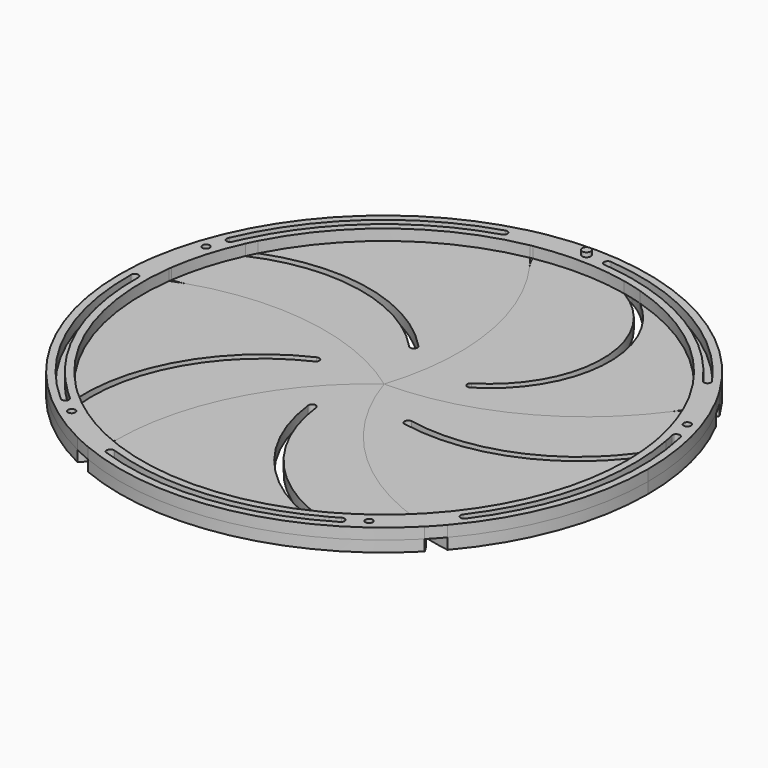
from build123d import *

# Parameters (mm, degrees)
F0_R     = 1.05
F1_DEPTH = 3.175
F2_DEPTH = 3.175
F3_DEPTH = 3.175
F4_DEPTH = 3.175
F5_DEPTH = 3.175
F6_DEPTH = 3.175
F7_R     = 1.05
F8_DEPTH = 25.4
F7_R_2   = 1.27
F9_DEPTH = 1.27


with BuildPart() as f1:
    # F0 (on Top) → F1 (new body)
    with BuildSketch(Plane.XY):
        with BuildLine():
            ThreePointArc((57.8988454356, -49.5395165219), (71.4784303906, -26.4059460899), (76.2, 0))
            ThreePointArc((76.2, 0), (74.0080436984, 18.1452326504), (67.5582816814, 35.2465399189))
            ThreePointArc((67.5582816814, 35.2465399189), (64.4660283996, 34.378247791), (61.6866117698, 32.7686500845))
            ThreePointArc((61.6866117698, 32.7686500846), (65.7907131471, 23.4649645981), (68.500497271, 13.6639808848))
            ThreePointArc((68.500497271, 13.6639808848), (69.3811022372, 15.2667591262), (70.201874573, 16.9009855397))
            ThreePointArc((70.201874573, 16.9009855397), (71.2638826106, 17.4908189825), (72.1717519503, 16.683640053))
            ThreePointArc((72.1717519503, 16.683640053), (72.2128589156, 16.5048063375), (72.2535227511, 16.3258713412))
            ThreePointArc((72.2535227511, 16.3258713412), (72.4179099959, -15.5804986063), (59.1463284149, -44.5961597006))
            ThreePointArc((59.1463284149, -44.5961597006), (57.6757970275, -44.802405764), (57.469550964, -43.3318743766))
            ThreePointArc((57.469550964, -43.3318743766), (70.0826247273, -16.3959243817), (70.727986059, 13.3398880445))
            ThreePointArc((70.727986059, 13.3398880445), (69.9127245645, 11.9184009517), (69.0527176616, 10.5235299949))
            ThreePointArc((69.0527176616, 10.5235299949), (69.6503942152, 5.2768442909), (69.85, 0))
            ThreePointArc((69.85, 0), (64.8935700225, -25.8427372725), (50.7276787478, -48.0179665215))
            ThreePointArc((50.7276787478, -48.0179665215), (54.2941569474, -48.8687853418), (57.8988454356, -49.5395165219))
        make_face()
        with Locations((69.4509021025, 22.5659660142)):
            Circle(F0_R, mode=Mode.SUBTRACT)
        with BuildLine():
            ThreePointArc((61.6866117698, 32.7686500845), (64.4660283996, 34.378247791), (67.5582816814, 35.2465399189))
            ThreePointArc((67.5582816814, 35.2465399189), (66.3207917987, 37.5232271425), (65.0066071965, 39.7565217391))
            ThreePointArc((65.0066071965, 39.7565217391), (63.2547939348, 36.5355265965), (61.3435147778, 33.4065217391))
            ThreePointArc((61.3435147778, 33.4065217391), (61.5158900581, 33.0880306208), (61.6866117698, 32.7686500846))
        make_face()
        with BuildLine():
            ThreePointArc((54.398108617, -53.359964195), (56.1809614325, -51.4795063352), (57.8988454356, -49.5395165219))
            ThreePointArc((57.8988454356, -49.5395165219), (54.2941569474, -48.8687853418), (50.7276787478, -48.0179665215))
            ThreePointArc((50.7276787478, -48.0179665215), (50.4780425853, -48.2803243232), (50.2270495554, -48.541384333))
            ThreePointArc((50.2270495554, -48.541384333), (52.6167549158, -50.6873735848), (54.398108617, -53.359964195))
        make_face()
        with BuildLine():
            ThreePointArc((61.3435147778, 33.4065217391), (63.2547939348, 36.5355265965), (65.0066071965, 39.7565217391))
            ThreePointArc((65.0066071965, 39.7565217391), (31.5990481128, 69.3393117817), (-12.6447943163, 75.1435238507))
            ThreePointArc((-12.6447943163, 75.1435238507), (-12.7745582452, 71.9342991933), (-12.1026268308, 68.7935238507))
            ThreePointArc((-12.1026268308, 68.7935238507), (1.2700549081, 69.8384525926), (14.5959016704, 68.3079948061))
            ThreePointArc((14.5959016704, 68.3079948061), (10.4665427153, 70.3209346952), (6.0938462702, 71.729145679))
            ThreePointArc((6.0938462702, 71.729145679), (5.3080441584, 72.9201009325), (6.4352132785, 73.7949432892))
            ThreePointArc((6.4352132785, 73.7949432892), (6.4752800387, 73.7914383477), (6.5153448899, 73.787911652))
            ThreePointArc((6.5153448899, 73.787911652), (37.0723258817, 64.1307124452), (60.69068892, 42.4705298226))
            ThreePointArc((60.69068892, 42.4705298226), (60.4324213932, 41.0082378256), (58.9701293962, 41.2665053524))
            ThreePointArc((58.9701293962, 41.2665053524), (39.869860882, 59.9232410526), (15.2829537028, 70.3337184508))
            ThreePointArc((15.2829537028, 70.3337184508), (17.9297919561, 68.6829049595), (20.4165739668, 66.799595863))
            ThreePointArc((20.4165739668, 66.799595863), (44.1582651124, 54.1208843448), (61.3435147778, 33.4065217391))
        make_face()
        with Locations((0, 73.025)):
            Circle(F0_R, mode=Mode.SUBTRACT)
        with BuildLine():
            ThreePointArc((-29.223152808, -70.3736267359), (15.1924579401, -74.6701360769), (54.398108617, -53.359964195))
            ThreePointArc((54.398108617, -53.359964195), (52.6167549158, -50.6873735848), (50.2270495554, -48.541384333))
            ThreePointArc((50.2270495554, -48.541384333), (42.6469559202, -55.3196136171), (34.1630358389, -60.9254419948))
            ThreePointArc((34.1630358389, -60.9254419949), (35.9594904295, -61.2676613714), (37.7673647093, -61.5432585154))
            ThreePointArc((37.7673647093, -61.5432585154), (38.6565081805, -62.3710196222), (38.1693824544, -63.4838866804))
            ThreePointArc((38.1693824544, -63.4838866804), (38.0120042348, -63.5782443848), (37.8543927568, -63.6722119453))
            ThreePointArc((37.8543927568, -63.6722119453), (7.5604301592, -73.6881640483), (-24.1362476499, -70.0324722852))
            ThreePointArc((-24.1362476499, -70.0324722852), (-24.7868185019, -68.6976473655), (-23.4519935822, -68.0470765134))
            ThreePointArc((-23.4519935822, -68.0470765134), (6.0632713273, -71.7191561984), (34.5431371215, -63.144059917))
            ThreePointArc((34.5431371215, -63.144059917), (32.9392929024, -62.8079638292), (31.3469350413, -62.4210874907))
            ThreePointArc((31.3469350413, -62.4210874907), (0.7540037914, -69.8459302915), (-29.9920851413, -63.0832571201))
            ThreePointArc((-29.9920851413, -63.0832571201), (-29.6991595508, -66.7380969266), (-29.223152808, -70.3736267359))
        make_face()
        with Locations((42.9230180487, -59.0784660142)):
            Circle(F0_R, mode=Mode.SUBTRACT)
        with BuildLine():
            ThreePointArc((-12.1026268308, 68.7935238507), (-12.7745582452, 71.9342991933), (-12.6447943163, 75.1435238507))
            ThreePointArc((-12.6447943163, 75.1435238507), (-15.1924579401, 74.6701360769), (-17.7225526948, 74.1103982311))
            ThreePointArc((-17.7225526948, 74.1103982311), (-15.2005443443, 71.4489825753), (-12.8153016257, 68.6643324022))
            ThreePointArc((-12.8153016257, 68.6643324022), (-12.4591316812, 68.7298518677), (-12.1026268308, 68.7935238507))
        make_face()
        with BuildLine():
            ThreePointArc((-33.9384016324, -68.2248114298), (-31.5990481128, -69.3393117817), (-29.223152808, -70.3736267359))
            ThreePointArc((-29.223152808, -70.3736267359), (-29.6991595508, -66.7380969266), (-29.9920851413, -63.0832571201))
            ThreePointArc((-29.9920851413, -63.0832571201), (-30.3187440548, -62.9269120404), (-30.6445879899, -62.7688754633))
            ThreePointArc((-30.6445879899, -62.7688754633), (-31.9470854839, -65.7047674669), (-33.9384016324, -68.2248114298))
        make_face()
        with BuildLine():
            ThreePointArc((-12.8153016257, 68.6643324022), (-15.2005443443, 71.4489825753), (-17.7225526948, 74.1103982311))
            ThreePointArc((-17.7225526948, 74.1103982311), (-56.1809614325, 51.4795063352), (-75.3731943497, 11.1947118553))
            ThreePointArc((-75.3731943497, 11.1947118553), (-72.3611395863, 10.0795940673), (-69.1664465044, 9.748085861))
            ThreePointArc((-69.1664465044, 9.748085861), (-67.0181651444, 19.6872557934), (-63.4495528671, 29.209189324))
            ThreePointArc((-63.4495528671, 29.209189324), (-65.1040666631, 28.4301211007), (-66.728659616, 27.590442034))
            ThreePointArc((-66.728659616, 27.590442034), (-67.9345375656, 27.7374894172), (-68.1945714194, 28.9241430976))
            ThreePointArc((-68.1945714194, 28.9241430976), (-68.1227118322, 29.0929846806), (-68.0504342143, 29.2616477363))
            ThreePointArc((-68.0504342143, 29.2616477363), (-49.4293325796, 55.1710676508), (-21.6374198617, 70.8443906511))
            ThreePointArc((-21.6374198617, 70.8443906511), (-20.3892075809, 70.305014085), (-20.7199588174, 68.9860885383))
            ThreePointArc((-20.7199588174, 68.9860885383), (-20.7480884716, 68.9666575811), (-20.7768358082, 68.948152712))
            ThreePointArc((-20.7768358082, 68.948152712), (-20.8967811774, 68.8840443635), (-21.0240066762, 68.8359772813))
            ThreePointArc((-21.0240066762, 68.8359772813), (-47.0607518656, 54.4581147199), (-65.0611321594, 30.7806709988))
            ThreePointArc((-65.0611321594, 30.7806709988), (-63.5660426061, 31.451479531), (-62.050397829, 32.0744544655))
            ThreePointArc((-62.050397829, 32.0744544655), (-41.664409639, 56.063352285), (-12.8153016257, 68.6643324022))
        make_face()
        with Locations((-69.4509021025, 22.5659660142)):
            Circle(F0_R, mode=Mode.SUBTRACT)
        with BuildLine():
            ThreePointArc((-75.9597471294, 6.0462232875), (-66.3207917987, -37.5232271425), (-33.9384016324, -68.2248114298))
            ThreePointArc((-33.9384016324, -68.2248114298), (-31.9470854839, -65.7047674669), (-30.6445879899, -62.7688754633))
            ThreePointArc((-30.6445879899, -62.7688754633), (-39.4334448718, -57.654366058), (-47.3865799637, -51.3179748173))
            ThreePointArc((-47.3865799637, -51.3179748173), (-47.1569149337, -53.132256265), (-46.8603595171, -54.9368110806))
            ThreePointArc((-46.8603595171, -54.9368110806), (-47.3728466687, -56.038229022), (-48.5817762639, -55.9188397594))
            ThreePointArc((-48.5817762639, -55.9188397594), (-48.720148318, -55.7983223123), (-48.8582214039, -55.6774624623))
            ThreePointArc((-48.8582214039, -55.6774624623), (-67.745307188, -29.9612913441), (-74.0633498234, 1.3137115121))
            ThreePointArc((-74.0633498234, 1.3137115121), (-72.9948933347, 2.344924745), (-71.9636801018, 1.2764682563))
            ThreePointArc((-71.9636801018, 1.2764682563), (-66.335316964, -27.9289517934), (-49.3791532399, -52.3650632608))
            ThreePointArc((-49.3791532399, -52.3650632608), (-49.5551219855, -50.7358573623), (-49.6792463629, -49.1018836789))
            ThreePointArc((-49.6792463629, -49.1018836789), (-66.1944271551, -22.3006796671), (-69.2638067586, 9.0303695003))
            ThreePointArc((-69.2638067586, 9.0303695003), (-72.6492469871, 7.6223730967), (-75.9597471294, 6.0462232875))
        make_face()
        with Locations((-42.9230180487, -59.0784660142)):
            Circle(F0_R, mode=Mode.SUBTRACT)
        with BuildLine():
            ThreePointArc((-69.1664465044, 9.748085861), (-72.3611395863, 10.0795940673), (-75.3731943497, 11.1947118553))
            ThreePointArc((-75.3731943497, 11.1947118553), (-75.7102471784, 8.6254548976), (-75.9597471294, 6.0462232875))
            ThreePointArc((-75.9597471294, 6.0462232875), (-72.6492469871, 7.6223730967), (-69.2638067586, 9.0303695003))
            ThreePointArc((-69.2638067586, 9.0303695003), (-69.2160569074, 9.3893538752), (-69.1664465044, 9.748085861))
        make_face()
        with BuildLine():
            ThreePointArc((-63.4495528671, 29.209189324), (-62.7663272963, 30.649806814), (-62.050397829, 32.0744544655))
            ThreePointArc((-62.050397829, 32.0744544655), (-63.5660426061, 31.451479531), (-65.0611321594, 30.7806709988))
            ThreePointArc((-65.0611321594, 30.7806709988), (-65.6748421089, 29.4485269405), (-66.2612794858, 28.1041538906))
            ThreePointArc((-66.2612794858, 28.1041538906), (-66.4512663757, 27.8075363811), (-66.728659616, 27.590442034))
            ThreePointArc((-66.728659616, 27.590442034), (-65.1040666631, 28.4301211007), (-63.4495528671, 29.209189324))
        make_face()
        with BuildLine():
            ThreePointArc((14.5959016704, 68.3079948061), (17.5224764061, 67.6164574686), (20.4165739668, 66.799595863))
            ThreePointArc((20.4165739668, 66.799595863), (17.9297919561, 68.6829049595), (15.2829537028, 70.3337184508))
            ThreePointArc((15.2829537028, 70.3337184508), (10.7896051737, 71.1616824225), (6.2527772625, 71.7028827977))
            ThreePointArc((6.2527772625, 71.7028827977), (6.1728073816, 71.7129619314), (6.0938462702, 71.729145679))
            ThreePointArc((6.0938462702, 71.729145679), (10.4665427153, 70.3209346952), (14.5959016704, 68.3079948061))
        make_face()
        with BuildLine():
            ThreePointArc((70.201874573, 16.9009855397), (69.3811022372, 15.2667591262), (68.500497271, 13.6639808848))
            ThreePointArc((68.500497271, 13.6639808848), (68.7945298881, 12.0969069385), (69.0527176616, 10.5235299949))
            ThreePointArc((69.0527176616, 10.5235299949), (69.9127245645, 11.9184009517), (70.727986059, 13.3398880445))
            ThreePointArc((70.727986059, 13.3398880445), (70.4414732064, 14.7783448841), (70.1257083581, 16.2106647697))
            ThreePointArc((70.1257083581, 16.2106647697), (70.105063583, 16.5623048678), (70.201874573, 16.9009855397))
        make_face()
        with BuildLine():
            ThreePointArc((37.7673647093, -61.5432585154), (35.9594904295, -61.2676613714), (34.1630358389, -60.9254419949))
            ThreePointArc((34.1630358389, -60.9254419948), (32.7635210263, -61.6893361121), (31.3469350413, -62.4210874907))
            ThreePointArc((31.3469350413, -62.4210874907), (32.9392929024, -62.8079638292), (34.5431371215, -63.144059917))
            ThreePointArc((34.5431371215, -63.144059917), (35.8226535316, -62.4270623925), (37.0872939879, -61.6841409898))
            ThreePointArc((37.0872939879, -61.6841409898), (37.4153440082, -61.5558438758), (37.7673647093, -61.5432585154))
        make_face()
        with BuildLine():
            ThreePointArc((-46.8603595171, -54.9368110806), (-47.1569149337, -53.132256265), (-47.3865799637, -51.3179748173))
            ThreePointArc((-47.3865799637, -51.3179748173), (-48.5455603027, -50.2230133992), (-49.6792463629, -49.1018836789))
            ThreePointArc((-49.6792463629, -49.1018836789), (-49.5551219855, -50.7358573623), (-49.3791532399, -52.3650632608))
            ThreePointArc((-49.3791532399, -52.3650632608), (-48.3018557566, -53.3603912604), (-47.2045001228, -54.3335604683))
            ThreePointArc((-47.2045001228, -54.3335604683), (-46.9811092852, -54.6059085892), (-46.8603595171, -54.9368110806))
        make_face()
    extrude(amount=F1_DEPTH)


with BuildPart() as f2:
    # F0 (on Top) → F2 (new body)
    with BuildSketch(Plane.XY):
        with BuildLine():
            ThreePointArc((61.3435147778, 33.4065217391), (63.2547939348, 36.5355265965), (65.0066071965, 39.7565217391))
            ThreePointArc((65.0066071965, 39.7565217391), (31.5990481128, 69.3393117817), (-12.6447943163, 75.1435238507))
            ThreePointArc((-12.6447943163, 75.1435238507), (-12.7745582452, 71.9342991933), (-12.1026268308, 68.7935238507))
            ThreePointArc((-12.1026268308, 68.7935238507), (1.2700549081, 69.8384525926), (14.5959016704, 68.3079948061))
            ThreePointArc((14.5959016704, 68.3079948061), (10.4665427153, 70.3209346952), (6.0938462702, 71.729145679))
            ThreePointArc((6.0938462702, 71.729145679), (5.3080441584, 72.9201009325), (6.4352132785, 73.7949432892))
            ThreePointArc((6.4352132785, 73.7949432892), (6.4752800387, 73.7914383477), (6.5153448899, 73.787911652))
            ThreePointArc((6.5153448899, 73.787911652), (37.0723258817, 64.1307124452), (60.69068892, 42.4705298226))
            ThreePointArc((60.69068892, 42.4705298226), (60.4324213932, 41.0082378256), (58.9701293962, 41.2665053524))
            ThreePointArc((58.9701293962, 41.2665053524), (39.869860882, 59.9232410526), (15.2829537028, 70.3337184508))
            ThreePointArc((15.2829537028, 70.3337184508), (17.9297919561, 68.6829049595), (20.4165739668, 66.799595863))
            ThreePointArc((20.4165739668, 66.799595863), (44.1582651124, 54.1208843448), (61.3435147778, 33.4065217391))
        make_face()
        with Locations((0, 73.025)):
            Circle(F0_R, mode=Mode.SUBTRACT)
        with BuildLine():
            ThreePointArc((59.0784660142, 30.1019819513), (60.2336563747, 31.7387157796), (61.3435147778, 33.4065217391))
            ThreePointArc((61.3435147778, 33.4065217391), (44.1582651124, 54.1208843448), (20.4165739668, 66.799595863))
            ThreePointArc((20.4165739668, 66.799595863), (32.7606539852, 37.7278540517), (16.2490976022, 10.8036829548))
            ThreePointArc((16.2490976022, 10.8036829548), (14.9772255674, 10.9446710874), (14.7861444758, 12.2099869147))
            ThreePointArc((14.7861444758, 12.2099869147), (14.9479136837, 12.4293059965), (15.160676558, 12.5996060128))
            ThreePointArc((15.160676558, 12.5996060128), (30.7540739017, 40.6147500395), (14.5959016704, 68.3079948061))
            ThreePointArc((14.5959016704, 68.3079948061), (1.2700549081, 69.8384525926), (-12.1026268308, 68.7935238507))
            ThreePointArc((-12.1026268308, 68.7935238507), (-11.3583497528, 67.0779959221), (-10.3724360882, 65.4889840629))
            ThreePointArc((-10.3724360882, 65.4889840629), (2.6750389695, 33.9895928238), (0, 0))
            ThreePointArc((0, 0), (33.1526562435, 7.9592485711), (59.0784660142, 30.1019819513))
        make_face()
        with BuildLine():
            ThreePointArc((6.5941442709, 73.7686804079), (11.055453508, 72.3469119056), (15.2829537028, 70.3337184508))
            ThreePointArc((15.2829537028, 70.3337184508), (39.869860882, 59.9232410526), (58.9701293962, 41.2665053524))
            ThreePointArc((58.9701293962, 41.2665053524), (60.4324213932, 41.0082378256), (60.69068892, 42.4705298226))
            ThreePointArc((60.69068892, 42.4705298226), (37.0723258817, 64.1307124452), (6.5153448899, 73.787911652))
            ThreePointArc((6.5153448899, 73.787911652), (6.5547502363, 73.7783192049), (6.5941442709, 73.7686804079))
        make_face()
    extrude(amount=-F2_DEPTH)


with BuildPart() as f2b:
    # F0 (on Top) → F2, piece 2 (new body)
    with BuildSketch(Plane.XY):
        with BuildLine():
            ThreePointArc((34.1630358389, -60.9254419948), (42.6469559202, -55.3196136171), (50.2270495554, -48.541384333))
            ThreePointArc((50.2270495554, -48.541384333), (48.6165547344, -47.5909681745), (46.8849360882, -46.8849360882))
            ThreePointArc((46.8849360882, -46.8849360882), (17.8144294063, -29.0705066819), (0, 0))
            ThreePointArc((0, 0), (-22.1427333802, -25.9258097708), (-30.1019819513, -59.0784660142))
            ThreePointArc((-30.1019819513, -59.0784660142), (-30.0745025786, -61.081615354), (-29.9920851413, -63.0832571201))
            ThreePointArc((-29.9920851413, -63.0832571201), (0.7540037914, -69.8459302915), (31.3469350413, -62.4210874907))
            ThreePointArc((31.3469350413, -62.4210874907), (5.5340708198, -46.501418093), (-6.8695410517, -18.826695952))
            ThreePointArc((-6.8695410517, -18.826695952), (-5.9562321753, -17.6558556998), (-4.7853919231, -18.5691645763))
            ThreePointArc((-4.7853919231, -18.5691645763), (7.8982881897, -45.9914925783), (34.1630358389, -60.9254419949))
        make_face()
    extrude(amount=-F2_DEPTH)

    # F0 (on Top) → F6 (join)
    with BuildSketch(Plane.XY):
        with BuildLine():
            ThreePointArc((37.8543927568, -63.6722119453), (36.1944718192, -63.4350516997), (34.5431371215, -63.144059917))
            ThreePointArc((34.5431371215, -63.144059917), (6.0632713273, -71.7191561984), (-23.4519935822, -68.0470765134))
            ThreePointArc((-23.4519935822, -68.0470765134), (-24.7868185019, -68.6976473655), (-24.1362476499, -70.0324722852))
            ThreePointArc((-24.1362476499, -70.0324722852), (7.5604301592, -73.6881640483), (37.8543927568, -63.6722119453))
        make_face()
        with BuildLine():
            ThreePointArc((-29.223152808, -70.3736267359), (15.1924579401, -74.6701360769), (54.398108617, -53.359964195))
            ThreePointArc((54.398108617, -53.359964195), (52.6167549158, -50.6873735848), (50.2270495554, -48.541384333))
            ThreePointArc((50.2270495554, -48.541384333), (42.6469559202, -55.3196136171), (34.1630358389, -60.9254419948))
            ThreePointArc((34.1630358389, -60.9254419949), (35.9594904295, -61.2676613714), (37.7673647093, -61.5432585154))
            ThreePointArc((37.7673647093, -61.5432585154), (38.6565081805, -62.3710196222), (38.1693824544, -63.4838866804))
            ThreePointArc((38.1693824544, -63.4838866804), (38.0120042348, -63.5782443848), (37.8543927568, -63.6722119453))
            ThreePointArc((37.8543927568, -63.6722119453), (7.5604301592, -73.6881640483), (-24.1362476499, -70.0324722852))
            ThreePointArc((-24.1362476499, -70.0324722852), (-24.7868185019, -68.6976473655), (-23.4519935822, -68.0470765134))
            ThreePointArc((-23.4519935822, -68.0470765134), (6.0632713273, -71.7191561984), (34.5431371215, -63.144059917))
            ThreePointArc((34.5431371215, -63.144059917), (32.9392929024, -62.8079638292), (31.3469350413, -62.4210874907))
            ThreePointArc((31.3469350413, -62.4210874907), (0.7540037914, -69.8459302915), (-29.9920851413, -63.0832571201))
            ThreePointArc((-29.9920851413, -63.0832571201), (-29.6991595508, -66.7380969266), (-29.223152808, -70.3736267359))
        make_face()
        with Locations((42.9230180487, -59.0784660142)):
            Circle(F0_R, mode=Mode.SUBTRACT)
        with BuildLine():
            ThreePointArc((34.1630358389, -60.9254419948), (42.6469559202, -55.3196136171), (50.2270495554, -48.541384333))
            ThreePointArc((50.2270495554, -48.541384333), (48.6165547344, -47.5909681745), (46.8849360882, -46.8849360882))
            ThreePointArc((46.8849360882, -46.8849360882), (17.8144294063, -29.0705066819), (0, 0))
            ThreePointArc((0, 0), (-22.1427333802, -25.9258097708), (-30.1019819513, -59.0784660142))
            ThreePointArc((-30.1019819513, -59.0784660142), (-30.0745025786, -61.081615354), (-29.9920851413, -63.0832571201))
            ThreePointArc((-29.9920851413, -63.0832571201), (0.7540037914, -69.8459302915), (31.3469350413, -62.4210874907))
            ThreePointArc((31.3469350413, -62.4210874907), (5.5340708198, -46.501418093), (-6.8695410517, -18.826695952))
            ThreePointArc((-6.8695410517, -18.826695952), (-5.9562321753, -17.6558556998), (-4.7853919231, -18.5691645763))
            ThreePointArc((-4.7853919231, -18.5691645763), (7.8982881897, -45.9914925783), (34.1630358389, -60.9254419949))
        make_face()
    extrude(amount=-F6_DEPTH)


with BuildPart() as f3:
    # F0 (on Top) → F3 (new body)
    with BuildSketch(Plane.XY):
        with BuildLine():
            ThreePointArc((68.500497271, 13.6639808848), (65.7907131471, 23.4649645981), (61.6866117698, 32.7686500846))
            ThreePointArc((61.6866117698, 32.7686500845), (60.2850420201, 31.5306732353), (59.0784660142, 30.1019819513))
            ThreePointArc((59.0784660142, 30.1019819513), (33.1526562435, 7.9592485711), (0, 0))
            ThreePointArc((0, 0), (17.8144294063, -29.0705066819), (46.8849360882, -46.8849360882))
            ThreePointArc((46.8849360882, -46.8849360882), (48.7985359141, -47.47780884), (50.7276787478, -48.0179665215))
            ThreePointArc((50.7276787478, -48.0179665215), (64.8935700225, -25.8427372725), (69.85, 0))
            ThreePointArc((69.85, 0), (69.6503942152, 5.2768442909), (69.0527176616, 10.5235299949))
            ThreePointArc((69.0527176616, 10.5235299949), (45.9355986257, -9.1065143384), (15.7824469369, -12.3510907783))
            ThreePointArc((15.7824469369, -12.3510907783), (14.9511396494, -11.1206728843), (16.1815575434, -10.2893655969))
            ThreePointArc((16.1815575434, -10.2893655969), (46.1812139878, -6.700434353), (68.500497271, 13.6639808848))
        make_face()
        with BuildLine():
            ThreePointArc((57.8988454356, -49.5395165219), (71.4784303906, -26.4059460899), (76.2, 0))
            ThreePointArc((76.2, 0), (74.0080436984, 18.1452326504), (67.5582816814, 35.2465399189))
            ThreePointArc((67.5582816814, 35.2465399189), (64.4660283996, 34.378247791), (61.6866117698, 32.7686500845))
            ThreePointArc((61.6866117698, 32.7686500846), (65.7907131471, 23.4649645981), (68.500497271, 13.6639808848))
            ThreePointArc((68.500497271, 13.6639808848), (69.3811022372, 15.2667591262), (70.201874573, 16.9009855397))
            ThreePointArc((70.201874573, 16.9009855397), (71.2638826106, 17.4908189825), (72.1717519503, 16.683640053))
            ThreePointArc((72.1717519503, 16.683640053), (72.2128589156, 16.5048063375), (72.2535227511, 16.3258713412))
            ThreePointArc((72.2535227511, 16.3258713412), (72.4179099959, -15.5804986063), (59.1463284149, -44.5961597006))
            ThreePointArc((59.1463284149, -44.5961597006), (57.6757970275, -44.802405764), (57.469550964, -43.3318743766))
            ThreePointArc((57.469550964, -43.3318743766), (70.0826247273, -16.3959243817), (70.727986059, 13.3398880445))
            ThreePointArc((70.727986059, 13.3398880445), (69.9127245645, 11.9184009517), (69.0527176616, 10.5235299949))
            ThreePointArc((69.0527176616, 10.5235299949), (69.6503942152, 5.2768442909), (69.85, 0))
            ThreePointArc((69.85, 0), (64.8935700225, -25.8427372725), (50.7276787478, -48.0179665215))
            ThreePointArc((50.7276787478, -48.0179665215), (54.2941569474, -48.8687853418), (57.8988454356, -49.5395165219))
        make_face()
        with Locations((69.4509021025, 22.5659660142)):
            Circle(F0_R, mode=Mode.SUBTRACT)
        with BuildLine():
            ThreePointArc((72.2535227511, 16.3258713412), (71.5150261751, 14.8204792632), (70.727986059, 13.3398880445))
            ThreePointArc((70.727986059, 13.3398880445), (70.0826247273, -16.3959243817), (57.469550964, -43.3318743766))
            ThreePointArc((57.469550964, -43.3318743766), (57.6757970275, -44.802405764), (59.1463284149, -44.5961597006))
            ThreePointArc((59.1463284149, -44.5961597006), (72.4179099959, -15.5804986063), (72.2535227511, 16.3258713412))
        make_face()
    extrude(amount=-F3_DEPTH)


with BuildPart() as f4:
    # F0 (on Top) → F4 (new body)
    with BuildSketch(Plane.XY):
        with BuildLine():
            ThreePointArc((-68.0504342143, 29.2616477363), (-66.5681306716, 30.0454581143), (-65.0611321594, 30.7806709988))
            ThreePointArc((-65.0611321594, 30.7806709988), (-47.0607518656, 54.4581147199), (-21.0240066762, 68.8359772813))
            ThreePointArc((-21.0240066762, 68.8359772813), (-20.8967811774, 68.8840443635), (-20.7768358082, 68.948152712))
            ThreePointArc((-20.7768358082, 68.948152712), (-20.7484067167, 68.9671347244), (-20.7199588174, 68.9860885383))
            ThreePointArc((-20.7199588174, 68.9860885383), (-20.3892075809, 70.305014085), (-21.6374198617, 70.8443906511))
            ThreePointArc((-21.6374198617, 70.8443906511), (-49.4293325796, 55.1710676508), (-68.0504342143, 29.2616477363))
        make_face()
        with BuildLine():
            ThreePointArc((-12.8153016257, 68.6643324022), (-15.2005443443, 71.4489825753), (-17.7225526948, 74.1103982311))
            ThreePointArc((-17.7225526948, 74.1103982311), (-56.1809614325, 51.4795063352), (-75.3731943497, 11.1947118553))
            ThreePointArc((-75.3731943497, 11.1947118553), (-72.3611395863, 10.0795940673), (-69.1664465044, 9.748085861))
            ThreePointArc((-69.1664465044, 9.748085861), (-67.0181651444, 19.6872557934), (-63.4495528671, 29.209189324))
            ThreePointArc((-63.4495528671, 29.209189324), (-65.1040666631, 28.4301211007), (-66.728659616, 27.590442034))
            ThreePointArc((-66.728659616, 27.590442034), (-67.9345375656, 27.7374894172), (-68.1945714194, 28.9241430976))
            ThreePointArc((-68.1945714194, 28.9241430976), (-68.1227118322, 29.0929846806), (-68.0504342143, 29.2616477363))
            ThreePointArc((-68.0504342143, 29.2616477363), (-49.4293325796, 55.1710676508), (-21.6374198617, 70.8443906511))
            ThreePointArc((-21.6374198617, 70.8443906511), (-20.3892075809, 70.305014085), (-20.7199588174, 68.9860885383))
            ThreePointArc((-20.7199588174, 68.9860885383), (-20.7480884716, 68.9666575811), (-20.7768358082, 68.948152712))
            ThreePointArc((-20.7768358082, 68.948152712), (-20.8967811774, 68.8840443635), (-21.0240066762, 68.8359772813))
            ThreePointArc((-21.0240066762, 68.8359772813), (-47.0607518656, 54.4581147199), (-65.0611321594, 30.7806709988))
            ThreePointArc((-65.0611321594, 30.7806709988), (-63.5660426061, 31.451479531), (-62.050397829, 32.0744544655))
            ThreePointArc((-62.050397829, 32.0744544655), (-41.664409639, 56.063352285), (-12.8153016257, 68.6643324022))
        make_face()
        with Locations((-69.4509021025, 22.5659660142)):
            Circle(F0_R, mode=Mode.SUBTRACT)
        with BuildLine():
            ThreePointArc((-65.4889840629, 10.3724360882), (-31.4993912391, 13.0474750577), (0, 0))
            ThreePointArc((0, 0), (2.6750389695, 33.9895928238), (-10.3724360882, 65.4889840629))
            ThreePointArc((-10.3724360882, 65.4889840629), (-11.5720890079, 67.093413951), (-12.8153016257, 68.6643324022))
            ThreePointArc((-12.8153016257, 68.6643324022), (-41.664409639, 56.063352285), (-62.050397829, 32.0744544655))
            ThreePointArc((-62.050397829, 32.0744544655), (-31.8100051071, 34.3675922868), (-5.5084787756, 19.2689318933))
            ThreePointArc((-5.5084787756, 19.2689318933), (-5.5591585447, 17.7848727432), (-7.0432176948, 17.8355525124))
            ThreePointArc((-7.0432176948, 17.8355525124), (-33.4229704404, 32.5654017762), (-63.4495528671, 29.209189324))
            ThreePointArc((-63.4495528671, 29.209189324), (-67.0181651444, 19.6872557934), (-69.1664465044, 9.748085861))
            ThreePointArc((-69.1664465044, 9.748085861), (-67.3048882234, 9.9258081418), (-65.4889840629, 10.3724360882))
        make_face()
    extrude(amount=-F4_DEPTH)


with BuildPart() as f5:
    # F0 (on Top) → F5 (new body)
    with BuildSketch(Plane.XY):
        with BuildLine():
            ThreePointArc((-48.8582214039, -55.6774624623), (-49.145612386, -54.0254972917), (-49.3791532399, -52.3650632608))
            ThreePointArc((-49.3791532399, -52.3650632608), (-66.335316964, -27.9289517934), (-71.9636801018, 1.2764682563))
            ThreePointArc((-71.9636801018, 1.2764682563), (-72.9948933347, 2.344924745), (-74.0633498234, 1.3137115121))
            ThreePointArc((-74.0633498234, 1.3137115121), (-67.745307188, -29.9612913441), (-48.8582214039, -55.6774624623))
        make_face()
        with BuildLine():
            ThreePointArc((-75.9597471294, 6.0462232875), (-66.3207917987, -37.5232271425), (-33.9384016324, -68.2248114298))
            ThreePointArc((-33.9384016324, -68.2248114298), (-31.9470854839, -65.7047674669), (-30.6445879899, -62.7688754633))
            ThreePointArc((-30.6445879899, -62.7688754633), (-39.4334448718, -57.654366058), (-47.3865799637, -51.3179748173))
            ThreePointArc((-47.3865799637, -51.3179748173), (-47.1569149337, -53.132256265), (-46.8603595171, -54.9368110806))
            ThreePointArc((-46.8603595171, -54.9368110806), (-47.3728466687, -56.038229022), (-48.5817762639, -55.9188397594))
            ThreePointArc((-48.5817762639, -55.9188397594), (-48.720148318, -55.7983223123), (-48.8582214039, -55.6774624623))
            ThreePointArc((-48.8582214039, -55.6774624623), (-67.745307188, -29.9612913441), (-74.0633498234, 1.3137115121))
            ThreePointArc((-74.0633498234, 1.3137115121), (-72.9948933347, 2.344924745), (-71.9636801018, 1.2764682563))
            ThreePointArc((-71.9636801018, 1.2764682563), (-66.335316964, -27.9289517934), (-49.3791532399, -52.3650632608))
            ThreePointArc((-49.3791532399, -52.3650632608), (-49.5551219855, -50.7358573623), (-49.6792463629, -49.1018836789))
            ThreePointArc((-49.6792463629, -49.1018836789), (-66.1944271551, -22.3006796671), (-69.2638067586, 9.0303695003))
            ThreePointArc((-69.2638067586, 9.0303695003), (-72.6492469871, 7.6223730967), (-75.9597471294, 6.0462232875))
        make_face()
        with Locations((-42.9230180487, -59.0784660142)):
            Circle(F0_R, mode=Mode.SUBTRACT)
        with BuildLine():
            ThreePointArc((-30.1019819513, -59.0784660142), (-22.1427333802, -25.9258097708), (0, 0))
            ThreePointArc((0, 0), (-31.4993912391, 13.0474750577), (-65.4889840629, 10.3724360882))
            ThreePointArc((-65.4889840629, 10.3724360882), (-67.3856007024, 9.7272944634), (-69.2638067586, 9.0303695003))
            ThreePointArc((-69.2638067586, 9.0303695003), (-66.1944271551, -22.3006796671), (-49.6792463629, -49.1018836789))
            ThreePointArc((-49.6792463629, -49.1018836789), (-42.5153547629, -19.6329425681), (-20.028056794, 0.7155527841))
            ThreePointArc((-20.028056794, 0.7155527841), (-18.6322935787, 0.2087539614), (-19.1390924014, -1.1870092539))
            ThreePointArc((-19.1390924014, -1.1870092539), (-41.2998034336, -21.7238712538), (-47.3865799637, -51.3179748173))
            ThreePointArc((-47.3865799637, -51.3179748173), (-39.4334448718, -57.654366058), (-30.6445879899, -62.7688754633))
            ThreePointArc((-30.6445879899, -62.7688754633), (-30.2383587783, -60.9435091246), (-30.1019819513, -59.0784660142))
        make_face()
    extrude(amount=-F5_DEPTH)


with BuildPart() as f8:
    # F7 (on face) → F8 (new body)
    with BuildSketch(Plane.XY.offset(3.175)):
        with Locations((0, 73.025)):
            Circle(F7_R)
    extrude(amount=-F8_DEPTH)

    # F7 (on face) → F9 (join)
    with BuildSketch(Plane.XY.offset(3.175)):
        with Locations((0, 73.025)):
            Circle(F7_R_2)
        with Locations((0, 73.025)):
            Circle(F7_R, mode=Mode.SUBTRACT)
        with Locations((0, 73.025)):
            Circle(F7_R)
    extrude(amount=F9_DEPTH)


solid = Compound([f1.part, f2.part, f2b.part, f3.part, f4.part, f5.part, f8.part])
